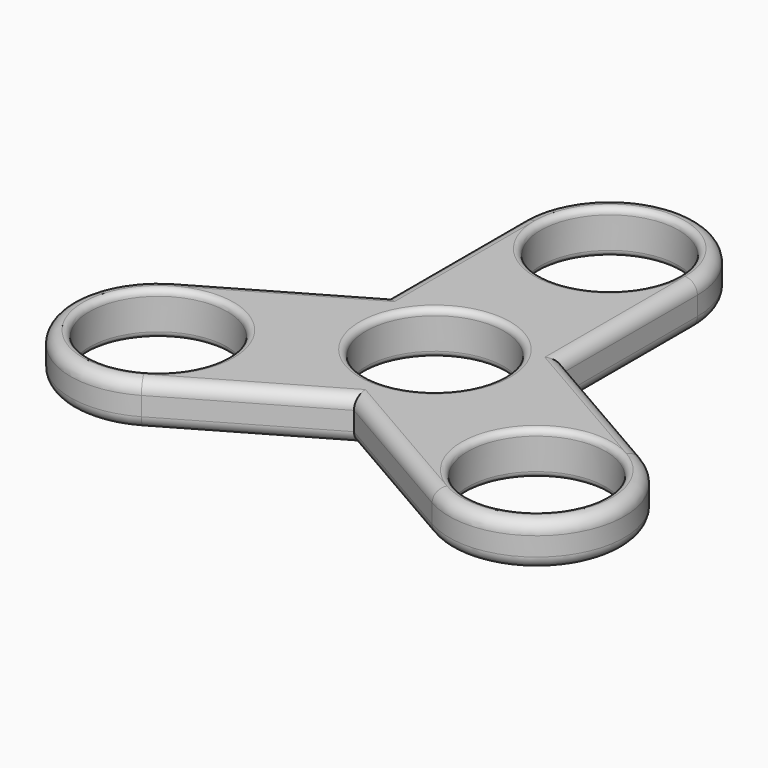
from build123d import *

# Parameters (mm, degrees)
F0_R     = 11.05
F1_DEPTH = 7
F2_COUNT = 3
F3_R     = 2
F4_R     = 0.99999


# Not quite as in the source:
# - a fillet or chamfer is up to 0.001 mm smaller than in the source, because OpenCascade refuses the exact size


with BuildPart() as f1:
    # F0 (on Top) → F1 (new body)
    with BuildSketch(Plane.XY):
        with BuildLine():
            Line((-14.05, 35), (-14.05, 0))
            ThreePointArc((-14.05, 0), (0, -14.05), (14.05, 0))
            Line((14.05, 0), (14.05, 35))
            ThreePointArc((14.05, 35), (0, 49.05), (-14.05, 35))
        make_face()
        Circle(F0_R, mode=Mode.SUBTRACT)
        with Locations((0, 35)):
            Circle(F0_R, mode=Mode.SUBTRACT)
    extrude(amount=F1_DEPTH)

    # F2: F1 ×3 about axis
    f2_axis = Axis((0, 0, 7), (0, 0, 1))


with BuildPart() as f1_1:
    add(f1.part)
    for i in range(1, F2_COUNT):
        add(f1.part.rotate(f2_axis, i * 360 / F2_COUNT))

    # F3
    f3_edges = [f1_1.edges().sort_by_distance(p)[0] for p in [
        (-25.692945, 1.389714, 0),
        (-14.05, 21.555886, 0),
        (25.692945, 1.389714, 0),
        (-25.692945, 1.389714, 7),
        (-14.05, 21.555886, 7),
        (11.642945, -22.9456, 7),
    ]]
    fillet(f3_edges, radius=F3_R)

    # F4 (radius 1 in the source; OpenCascade refuses exactly that, so slightly less here)
    f4_edges = [f1_1.edges().sort_by_distance(p)[0] for p in [
        (-24.785889, -27.069581, 0),
        (-24.785889, -27.069581, 7),
        (-11.05, 0, 0),
        (-11.05, 0, 7),
        (-11.05, 35, 0),
        (-11.05, 35, 7),
        (35.835889, -7.930419, 0),
        (35.835889, -7.930419, 7),
    ]]
    fillet(f4_edges, radius=F4_R)


solid = f1_1.part
